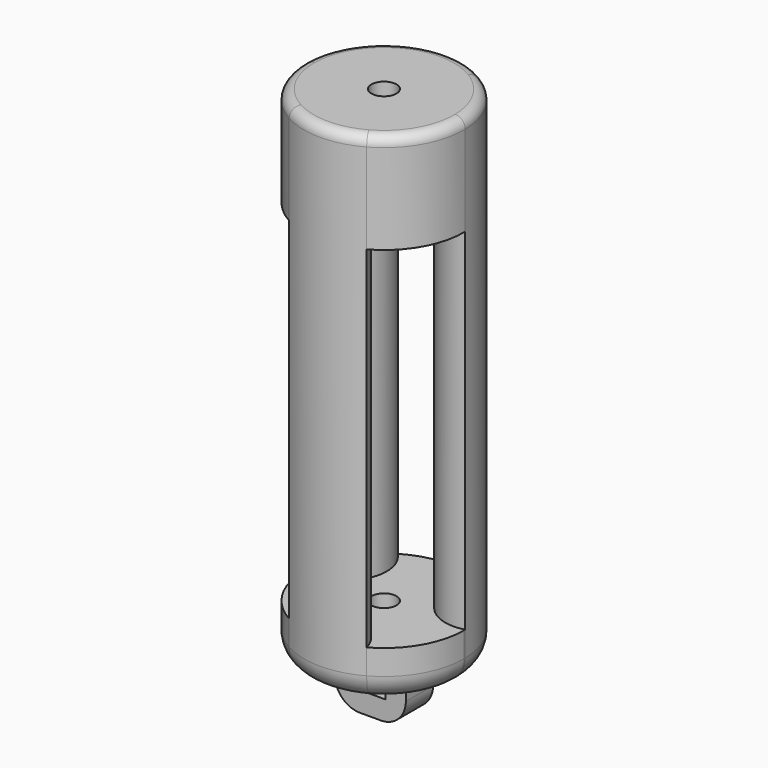
from build123d import *

# Parameters (mm, degrees)
F1_DEPTH     = 10
F2_DEPTH     = 70
F4_DEPTH     = 20
F6_D         = 5
F8_DEPTH     = 5
F9_W         = 4.088002
F9_H         = 6.796502
F9_W_2       = 10.088002
F10_DEPTH    = 4
F11_T1_DEPTH = 31.796502
F12_R        = 2
F13_R        = 5


# Not quite as in the source:
# - a fillet or chamfer that OpenCascade refuses, or shapes differently, is made with other operations: its cross-section is extruded or revolved along the edge and cut away or added


with BuildPart() as f1:
    # F0 (on Top) → F1 (new body)
    with BuildSketch(Plane.XY):
        with BuildLine():
            ThreePointArc((7.745967, -14), (13.782878, -8.126024), (16, 0))
            ThreePointArc((16, 0), (15.999335, 0.145904), (15.997339, 0.291796))
            ThreePointArc((15.997339, 0.291796), (6.928203, 4), (8.251372, 13.708204))
            ThreePointArc((8.251372, 13.708204), (0, 16), (-8.251372, 13.708204))
            ThreePointArc((-8.251372, 13.708204), (-6.928203, 4), (-15.997339, 0.291796))
            ThreePointArc((-15.997339, 0.291796), (-13.856406, -8), (-7.745967, -14))
            ThreePointArc((-7.745967, -14), (0, -8), (7.745967, -14))
        make_face()
        with BuildLine():
            ThreePointArc((-15.997339, 0.291796), (-6.928203, 4), (-8.251372, 13.708204))
            ThreePointArc((-8.251372, 13.708204), (-13.856406, 8), (-15.997339, 0.291796))
        make_face()
        with BuildLine():
            ThreePointArc((8.251372, 13.708204), (6.928203, 4), (15.997339, 0.291796))
            ThreePointArc((15.997339, 0.291796), (13.856406, 8), (8.251372, 13.708204))
        make_face()
        with BuildLine():
            ThreePointArc((-7.745967, -14), (0, -16), (7.745967, -14))
            ThreePointArc((7.745967, -14), (0, -8), (-7.745967, -14))
        make_face()
    extrude(amount=-F1_DEPTH)

    # F0 (on Top) → F2 (join)
    with BuildSketch(Plane.XY):
        with BuildLine():
            ThreePointArc((-15.997339, 0.291796), (-6.928203, 4), (-8.251372, 13.708204))
            ThreePointArc((-8.251372, 13.708204), (-13.856406, 8), (-15.997339, 0.291796))
        make_face()
        with BuildLine():
            ThreePointArc((8.251372, 13.708204), (6.928203, 4), (15.997339, 0.291796))
            ThreePointArc((15.997339, 0.291796), (13.856406, 8), (8.251372, 13.708204))
        make_face()
        with BuildLine():
            ThreePointArc((-7.745967, -14), (0, -16), (7.745967, -14))
            ThreePointArc((7.745967, -14), (0, -8), (-7.745967, -14))
        make_face()
    extrude(amount=F2_DEPTH)

    # F3 (on face) + F2_face (on face) → F4 (join)
    with BuildSketch(Plane.XY.offset(70)):
        with BuildLine():
            ThreePointArc((-15.997339, 0.291796), (-13.856406, -8), (-7.745967, -14))
            ThreePointArc((-7.745967, -14), (0, -8), (7.745967, -14))
            ThreePointArc((7.745967, -14), (13.856406, -8), (15.997339, 0.291796))
            ThreePointArc((15.997339, 0.291796), (6.928203, 4), (8.251372, 13.708204))
            ThreePointArc((8.251372, 13.708204), (0, 16), (-8.251372, 13.708204))
            ThreePointArc((-8.251372, 13.708204), (-6.928203, 4), (-15.997339, 0.291796))
        make_face()
        with BuildLine():
            ThreePointArc((7.745967, -14), (0, -8), (-7.745967, -14))
            ThreePointArc((-7.745967, -14), (0, -16), (7.745967, -14))
        make_face()
    with BuildSketch(Plane(origin=(0, -12.27089, 70), x_dir=(1, 0, 0), z_dir=(0, 0, 1))):
        with BuildLine():
            ThreePointArc((-15.997339, 12.562686), (-6.928203, 16.27089), (-8.251372, 25.979094))
            ThreePointArc((-8.251372, 25.979094), (-13.856406, 20.27089), (-15.997339, 12.562686))
        make_face()
        with BuildLine():
            ThreePointArc((8.251372, 25.979094), (6.928203, 16.27089), (15.997339, 12.562686))
            ThreePointArc((15.997339, 12.562686), (13.856406, 20.27089), (8.251372, 25.979094))
        make_face()
    extrude(amount=F4_DEPTH)

    # F6 (through all)
    with Locations(Plane.XY.offset(90)):
        with Locations((0, 0)):
            Hole(F6_D / 2)

    # F7 (on face) → F8 (join)
    with BuildSketch(Plane(origin=(0, 0, -10), x_dir=(1, 0, 0), z_dir=(0, 0, -1))):
        Polygon((-3, -3.398251), (-3, 3.398251), (-7.088002, 3.398251), (-7.088002, 0), (-7.088002, -3.398251), align=None)
        Polygon((7.088002, 3.398251), (3, 3.398251), (3, -3.398251), (7.088002, -3.398251), (7.088002, 0), align=None)
    extrude(amount=F8_DEPTH)

    # F9 (on face) → F10 (join)
    with BuildSketch(Plane(origin=(0, 0, -15), x_dir=(1, 0, 0), z_dir=(0, 0, -1))):
        with Locations((-5.044001, 0)):
            Rectangle(F9_W, F9_H)
        with Locations((2.044001, 0)):
            Rectangle(F9_W_2, F9_H)
    extrude(amount=F10_DEPTH)

    # F11: fillet of radius 5 on 2 edges, made by hand

    # F11_s2 → F11_t1 (cut)
    with BuildSketch(Plane.XZ.offset(-15.898251)):
        with BuildLine():
            ThreePointArc((-7.088002, -14), (-5.623536, -17.535534), (-2.088002, -19))
            Line((-2.088002, -19), (-7.088002, -19))
            Line((-7.088002, -19), (-7.088002, -14))
        make_face()
        with BuildLine():
            ThreePointArc((7.088002, -14), (5.623536, -17.535534), (2.088002, -19))
            Line((2.088002, -19), (7.088002, -19))
            Line((7.088002, -19), (7.088002, -14))
        make_face()
    extrude(amount=F11_T1_DEPTH, mode=Mode.SUBTRACT)

    # F12
    f12_edges = [f1.edges().sort_by_distance(p)[0] for p in [
        (-15.997339, -0.291796, 90),
    ]]
    fillet(f12_edges, radius=F12_R)

    # F13
    f13_edges = [f1.edges().sort_by_distance(p)[0] for p in [
        (7.745967, 14, -10),
    ]]
    fillet(f13_edges, radius=F13_R)


solid = f1.part
